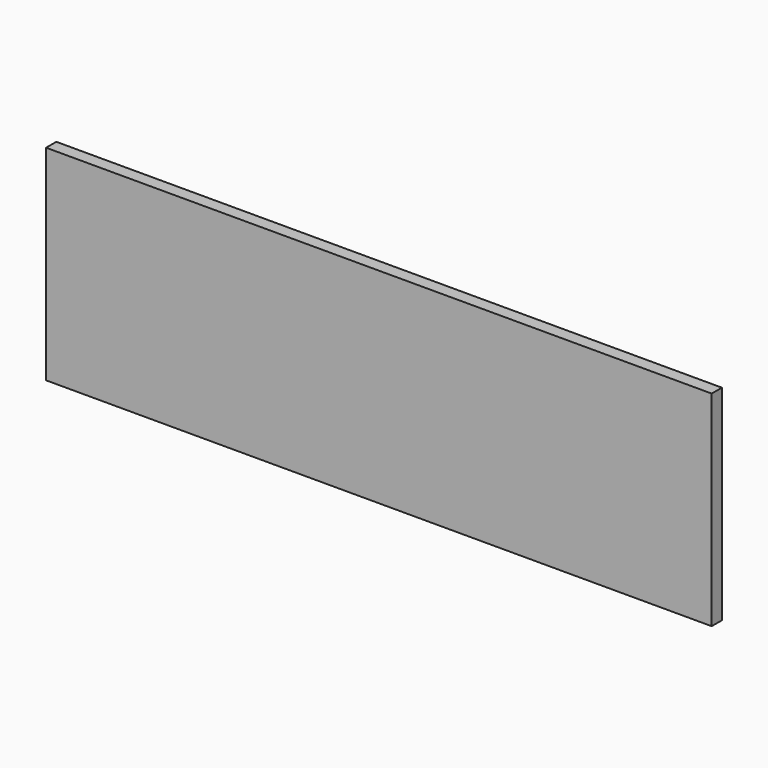
from build123d import *

# Parameters (mm, degrees)
F0_W     = 165.1
F0_H     = 50.8
F1_DEPTH = 3.175


# Not quite as in the source:
# - a length typed as a fraction of an inch, garbled in the dataset ("3 / 203.2 mm" for 3/8 in), is restored


with BuildPart() as f1:
    # F0 (on Front) → F1 (new body)
    with BuildSketch(Plane.XZ):
        with Locations((-82.55, 25.4)):
            Rectangle(F0_W, F0_H)
    extrude(amount=F1_DEPTH)


solid = f1.part
